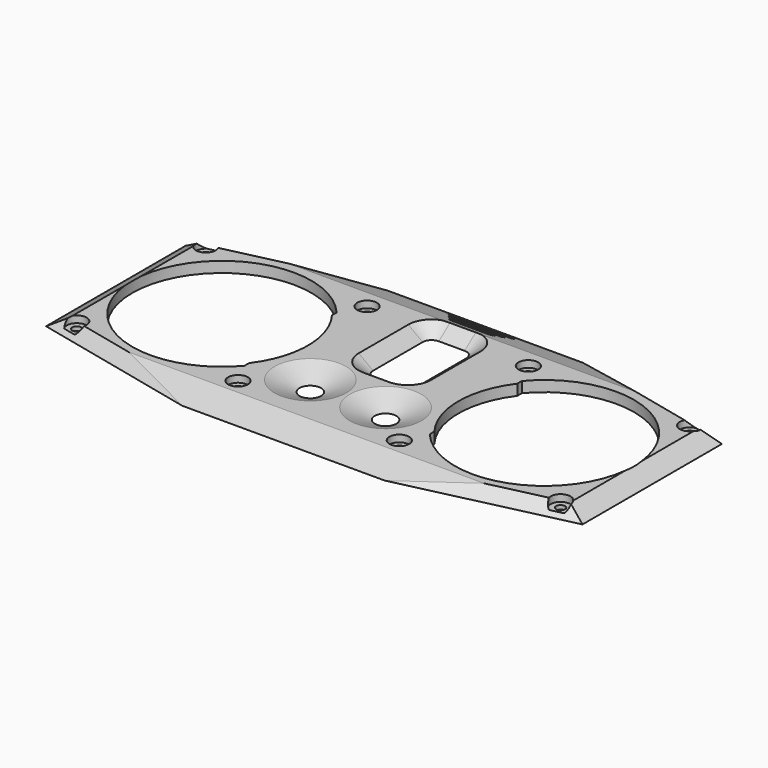
from build123d import *

# Parameters (mm, degrees)
F0_R        = 1.25
F0_R_2      = 3
F1_DEPTH    = 3
F2_SIZE2    = 6.99999
F2_SIZE     = 2.99999
F2_2_SIZE2  = 6.99999
F2_2_SIZE   = 2.99999
F3_SIZE2    = 2.99999
F3_SIZE     = 3.99999
F4_T1_DEPTH = 178.8917354422
F4_T3_DEPTH = 181.0057878677
F5_T1_DEPTH = 74.4931306538
F6_T1_DEPTH = 53.4058582454
F6_T3_DEPTH = 54.4906885897
F6_T5_DEPTH = 53.4058582454
F6_T7_DEPTH = 54.4906885841
F7_R        = 2.75
F7_R_2      = 1.25
F8_DEPTH    = 1.9


# Not quite as in the source:
# - a fillet or chamfer that OpenCascade refuses, or shapes differently, is made with other operations: its cross-section is extruded or revolved along the edge and cut away or added
# - a fillet or chamfer is up to 0.001 mm smaller than in the source, because OpenCascade refuses the exact size


with BuildPart() as f1:
    # F0 (on Top) → F1 (new body)
    with BuildSketch(Plane.XY):
        Polygon((-44.1484891925, -17.5328822659), (-29.4527173684, -20.9256685242), (27.0472826316, -20.9256685242), (73.6322826316, -10.1706738406), (73.6322826316, 38.4598458413), (25.9902564184, 49.4588742547), (-28.3956911556, 49.4588742546), (-76.037717368, 38.4598458414), (-76.0377173684, -10.1706738406), align=None)
        with Locations((-68.7027173684, -8.6404804453)):
            Circle(F0_R, mode=Mode.SUBTRACT)
        with Locations((-23.7027173684, -8.6404804453)):
            Circle(F0_R, mode=Mode.SUBTRACT)
        with BuildLine():
            ThreePointArc((-27.0502267204, -2.2085264366), (-71.2027173684, 13.8595195547), (-27.0502267204, 29.927565546))
            Line((-27.0502267204, 29.927565546), (-27.0502267204, 28.3226486068))
            ThreePointArc((-27.0502267204, 28.3226486068), (-22.2027173684, 13.8595195547), (-27.0502267204, -0.6036094974))
            Line((-27.0502267204, -0.6036094974), (-27.0502267204, -2.2085264366))
        make_face(mode=Mode.SUBTRACT)
        with Locations((-11.7027286338, 1.5743587088)):
            Circle(F0_R_2, mode=Mode.SUBTRACT)
        with Locations((21.2972826316, -8.6404804453)):
            Circle(F0_R, mode=Mode.SUBTRACT)
        with Locations((66.2972826316, -8.6404804453)):
            Circle(F0_R, mode=Mode.SUBTRACT)
        with Locations((9.2972956984, 1.5743587088)):
            Circle(F0_R_2, mode=Mode.SUBTRACT)
        with BuildLine():
            ThreePointArc((24.6447919836, 29.927565546), (68.7972826316, 13.8595195547), (24.6447919836, -2.2085264366))
            Line((24.6447919836, -2.2085264366), (24.6447919836, -0.6036094974))
            ThreePointArc((24.6447919836, -0.6036094974), (19.7972826316, 13.8595195547), (24.6447919836, 28.3226486068))
            Line((24.6447919836, 28.3226486068), (24.6447919836, 29.927565546))
        make_face(mode=Mode.SUBTRACT)
        with BuildLine():
            Line((4.8972822306, 35.2537547127), (4.8972822306, 17.9537547127))
            ThreePointArc((4.8972822306, 17.9537547127), (4.1650491836, 16.1859877597), (2.3972822306, 15.4537547127))
            Line((2.3972822306, 15.4537547127), (-4.8027177694, 15.4537547127))
            ThreePointArc((-4.8027177694, 15.4537547127), (-6.5704847223, 16.1859877597), (-7.3027177694, 17.9537547127))
            Line((-7.3027177694, 17.9537547127), (-7.3027177694, 35.2537547127))
            ThreePointArc((-7.3027177694, 35.2537547127), (-6.5704847223, 37.0215216656), (-4.8027177694, 37.7537547127))
            Line((-4.8027177694, 37.7537547127), (2.3972822306, 37.7537547127))
            ThreePointArc((2.3972822306, 37.7537547127), (4.1650491836, 37.0215216656), (4.8972822306, 35.2537547127))
        make_face(mode=Mode.SUBTRACT)
        with Locations((-68.7027173684, 36.3595195547)):
            Circle(F0_R, mode=Mode.SUBTRACT)
        with Locations((-23.7027173684, 36.3595195547)):
            Circle(F0_R, mode=Mode.SUBTRACT)
        Polygon((-7.7027173684, 44.858563391), (5.2972826316, 44.858563391), (4.4972826316, 44.058563391), (-6.9027173684, 44.058563391), align=None, mode=Mode.SUBTRACT)
        Polygon((-9.2027173684, 46.658563391), (6.7972826316, 46.658563391), (5.9972826316, 45.858563391), (-8.4027173684, 45.858563391), align=None, mode=Mode.SUBTRACT)
        Polygon((-10.7027173684, 48.458563391), (8.2972826316, 48.458563391), (7.4972826316, 47.658563391), (-9.9027173684, 47.658563391), align=None, mode=Mode.SUBTRACT)
        with Locations((21.2972826316, 36.3595195547)):
            Circle(F0_R, mode=Mode.SUBTRACT)
        with Locations((66.2972826316, 36.3595195547)):
            Circle(F0_R, mode=Mode.SUBTRACT)
    extrude(amount=F1_DEPTH)

    # F2 (size 3 and 7 in the source; OpenCascade refuses exactly that, so slightly less here)
    f2_edges = [f1.edges().sort_by_distance(p)[0] for p in [
        (6.297296, 1.574359, 3),
    ]]
    f2_side = f1.faces().sort_by_distance((6.297296, 1.574359, 1.5))[0]
    chamfer(f2_edges, length=F2_SIZE, length2=F2_SIZE2, reference=f2_side)

    # F2#2 (size 3 and 7 in the source; OpenCascade refuses exactly that, so slightly less here)
    f2_2_edges = [f1.edges().sort_by_distance(p)[0] for p in [
        (-14.702729, 1.574359, 3),
    ]]
    f2_2_side = f1.faces().sort_by_distance((-14.702729, 1.574359, 1.5))[0]
    chamfer(f2_2_edges, length=F2_2_SIZE, length2=F2_2_SIZE2, reference=f2_2_side)

    # F3 (size 4 and 3 in the source; OpenCascade refuses exactly that, so slightly less here)
    f3_edges = [f1.edges().sort_by_distance(p)[0] for p in [
        (-1.202718, 37.753755, 3),
        (-7.302718, 26.603755, 3),
        (-1.202718, 15.453755, 3),
        (-6.570485, 16.185988, 3),
        (4.165049, 16.185988, 3),
        (4.897282, 26.603755, 3),
        (4.165049, 37.021522, 3),
        (-6.570485, 37.021522, 3),
    ]]
    f3_side = f1.faces().sort_by_distance((-1.202717, 15.209837, 3))[0]
    chamfer(f3_edges, length=F3_SIZE, length2=F3_SIZE2, reference=f3_side)

    # F4: chamfer of 3 x 8 on 2 edges, made by hand

    # F4_s2 → F4_t1 (cut)
    with BuildSketch(Plane.YZ.offset(-90.6485850894)):
        Polygon((41.4588742546, 3), (49.4588742546, 0), (49.4588742546, 3), align=None)
    extrude(amount=F4_T1_DEPTH, mode=Mode.SUBTRACT)

    # F4_s4 → F4_t3 (cut)
    with BuildSketch(Plane.YZ.offset(-91.7056113022)):
        Polygon((-12.9256685242, 3), (-20.9256685242, 0), (-20.9256685242, 3), align=None)
    extrude(amount=F4_T3_DEPTH, mode=Mode.SUBTRACT)

    # F5: chamfer of 5 x 3 on 2 edges, made by hand

    # F5_s2 → F5_t1 (cut)
    with BuildSketch(Plane.XZ.offset(-51.3911513272)):
        Polygon((-71.0377173684, 3), (-76.0377173684, 0), (-76.0377173684, 3), align=None)
        Polygon((68.6322826316, 3), (73.6322826316, 0), (73.6322826316, 3), align=None)
    extrude(amount=F5_T1_DEPTH, mode=Mode.SUBTRACT)

    # F6: chamfer of 3 on 4 edges, made by hand

    # F6_s2 → F6_t1 (cut)
    with BuildSketch(Plane(origin=(-20.4409607394, 4.7191676308, 0), x_dir=(0, 0, 1), z_dir=(-0.9743700648, 0.2249510543, 0))):
        Polygon((3, -24.0147648209), (0, -27.0147648209), (3, -27.0147648209), align=None)
    extrude(amount=F6_T1_DEPTH, mode=Mode.SUBTRACT)

    # F6_s4 → F6_t3 (cut)
    with BuildSketch(Plane(origin=(-13.1833561407, -3.0436175852, 0), x_dir=(0, 0, 1), z_dir=(-0.9743700648, -0.2249510543, 0))):
        Polygon((3, 51.5788871759), (0, 54.5788871759), (3, 54.5788871759), align=None)
    extrude(amount=F6_T3_DEPTH, mode=Mode.SUBTRACT)

    # F6_s6 → F6_t5 (cut)
    with BuildSketch(Plane(origin=(18.1572481609, 4.1919310387, 0), x_dir=(0, 0, 1), z_dir=(0.9743700648, 0.2249510543, 0))):
        Polygon((3, 23.4736597407), (0, 26.4736597407), (3, 26.4736597407), align=None)
    extrude(amount=F6_T5_DEPTH, mode=Mode.SUBTRACT)

    # F6_s8 → F6_t7 (cut)
    with BuildSketch(Plane(origin=(63.9937393355, -14.7741188415, 0), x_dir=(0, 0, 1), z_dir=(-0.9743700648, 0.2249510543, 0))):
        Polygon((3, 51.0377820952), (0, 54.0377820952), (3, 54.0377820952), align=None)
    extrude(amount=F6_T7_DEPTH, mode=Mode.SUBTRACT)

    # F7 (on face) → F8 (cut)
    with BuildSketch(Plane.XY.offset(3)):
        with Locations((-68.7027173684, 36.3595195547)):
            Circle(F7_R)
        with Locations((-68.7027173684, 36.3595195547)):
            Circle(F7_R_2, mode=Mode.SUBTRACT)
        with Locations((-23.7027173684, 36.3595195547)):
            Circle(F7_R)
        with Locations((-23.7027173684, 36.3595195547)):
            Circle(F7_R_2, mode=Mode.SUBTRACT)
        with Locations((21.2972826316, 36.3595195547)):
            Circle(F7_R)
        with Locations((21.2972826316, 36.3595195547)):
            Circle(F7_R_2, mode=Mode.SUBTRACT)
        with Locations((66.2972826316, 36.3595195547)):
            Circle(F7_R)
        with Locations((66.2972826316, 36.3595195547)):
            Circle(F7_R_2, mode=Mode.SUBTRACT)
        with Locations((66.2972826316, -8.6404804453)):
            Circle(F7_R)
        with Locations((66.2972826316, -8.6404804453)):
            Circle(F7_R_2, mode=Mode.SUBTRACT)
        with Locations((21.2972826316, -8.6404804453)):
            Circle(F7_R)
        with Locations((21.2972826316, -8.6404804453)):
            Circle(F7_R_2, mode=Mode.SUBTRACT)
        with Locations((-23.7027173684, -8.6404804453)):
            Circle(F7_R)
        with Locations((-23.7027173684, -8.6404804453)):
            Circle(F7_R_2, mode=Mode.SUBTRACT)
        with Locations((-68.7027173684, -8.6404804453)):
            Circle(F7_R)
        with Locations((-68.7027173684, -8.6404804453)):
            Circle(F7_R_2, mode=Mode.SUBTRACT)
    extrude(amount=-F8_DEPTH, mode=Mode.SUBTRACT)


solid = f1.part
